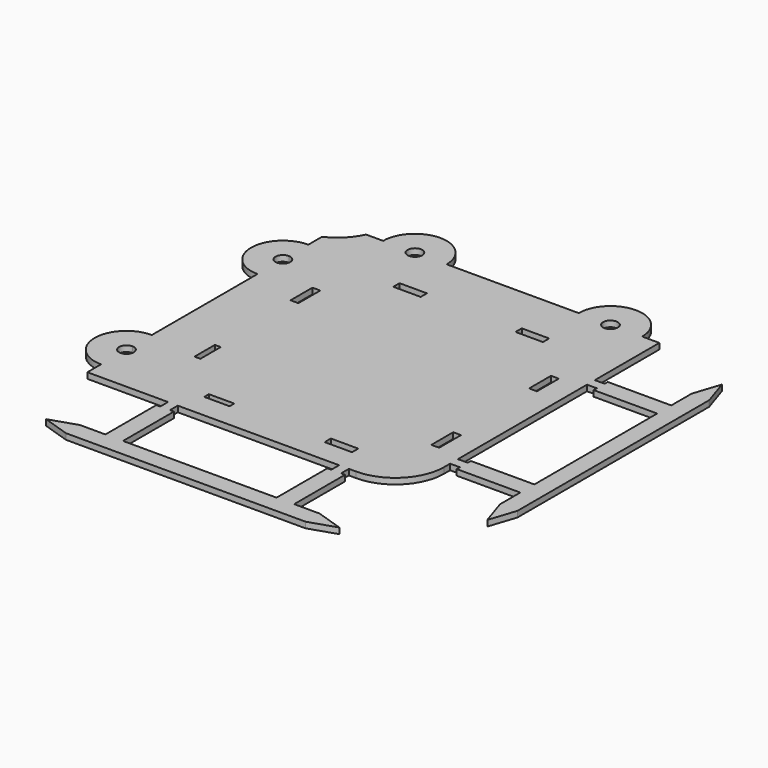
from build123d import *

# Parameters (mm, degrees)
F0_R        = 1.905
F0_W        = 2.032
F0_H        = 7.112
F0_W_2      = 7.112
F0_H_2      = 2.032
F0_W_3      = 2.54
F0_H_3      = 2.54
F0_W_4      = 6.604
F0_H_4      = 1.524
F0_W_5      = 1.524
F0_H_5      = 6.604
F1_DEPTH    = 1.524
F2_T1_DEPTH = 1.524
F2_T3_DEPTH = 65.024


# Not quite as in the source:
# - a fillet or chamfer that OpenCascade refuses, or shapes differently, is made with other operations: its cross-section is extruded or revolved along the edge and cut away or added


with BuildPart() as f1:
    # F0 (on Top) → F1 (new body)
    with BuildSketch(Plane.XY):
        with BuildLine():
            Line((38.1, 23.495), (38.1, 38.1))
            Line((38.1, 38.1), (30.674706153, 38.1))
            ThreePointArc((30.674706153, 38.1), (25.4, 36.195), (20.125293847, 38.1))
            Line((20.125293847, 38.1), (-20.125293847, 38.1))
            ThreePointArc((-20.125293847, 38.1), (-25.4, 36.195), (-30.674706153, 38.1))
            Line((-30.674706153, 38.1), (-38.1, 38.1))
            Line((-38.1, 38.1), (-38.1, 30.674706153))
            ThreePointArc((-38.1, 30.674706153), (-36.6858427695, 28.2040840751), (-36.195, 25.4))
            ThreePointArc((-36.195, 25.4), (-36.6858427695, 22.5959159249), (-38.1, 20.125293847))
            Line((-38.1, 20.125293847), (-38.1, -20.125293847))
            ThreePointArc((-38.1, -20.125293847), (-36.6858427695, -22.5959159249), (-36.195, -25.4))
            ThreePointArc((-36.195, -25.4), (-36.6858427695, -28.2040840751), (-38.1, -30.674706153))
            Line((-38.1, -30.674706153), (-38.1, -38.1))
            Line((-38.1, -38.1), (-23.495, -38.1))
            Line((-23.495, -38.1), (-20.955, -38.1))
            Line((-20.955, -38.1), (20.955, -38.1))
            Line((20.955, -38.1), (23.495, -38.1))
            Line((23.495, -38.1), (38.1, -38.1))
            Line((38.1, -38.1), (38.1, -23.495))
            Line((38.1, -23.495), (38.1, -20.955))
            Line((38.1, -20.955), (38.1, 20.955))
            Line((38.1, 20.955), (38.1, 23.495))
        make_face()
        with Locations((-25.4, -25.4)):
            Circle(F0_R, mode=Mode.SUBTRACT)
        with Locations((-30.988, -15.875)):
            Rectangle(F0_W, F0_H, mode=Mode.SUBTRACT)
        with Locations((-15.875, -30.988)):
            Rectangle(F0_W_2, F0_H_2, mode=Mode.SUBTRACT)
        with Locations((15.875, -30.988)):
            Rectangle(F0_W_2, F0_H_2, mode=Mode.SUBTRACT)
        with Locations((25.4, -25.4)):
            Circle(F0_R, mode=Mode.SUBTRACT)
        with Locations((30.988, -15.875)):
            Rectangle(F0_W, F0_H, mode=Mode.SUBTRACT)
        with Locations((-30.988, 15.875)):
            Rectangle(F0_W, F0_H, mode=Mode.SUBTRACT)
        with Locations((-25.4, 25.4)):
            Circle(F0_R, mode=Mode.SUBTRACT)
        with Locations((-15.875, 30.988)):
            Rectangle(F0_W_2, F0_H_2, mode=Mode.SUBTRACT)
        with Locations((30.988, 15.875)):
            Rectangle(F0_W, F0_H, mode=Mode.SUBTRACT)
        with Locations((15.875, 30.988)):
            Rectangle(F0_W_2, F0_H_2, mode=Mode.SUBTRACT)
        with Locations((25.4, 25.4)):
            Circle(F0_R, mode=Mode.SUBTRACT)
        Polygon((31.1238057911, -57.15), (24.511, -57.15), (19.939, -57.15), (0, -57.15), (-19.939, -57.15), (-24.511, -57.15), (-31.1238057911, -57.15), (-38.1, -59.436), (-31.1238057911, -61.722), (0, -61.722), (31.1238057911, -61.722), (38.1, -59.436), align=None)
        Polygon((-19.939, -40.64), (-20.955, -40.64), (-23.495, -40.64), (-24.511, -40.64), (-24.511, -57.15), (-19.939, -57.15), align=None)
        Polygon((24.511, -40.64), (23.495, -40.64), (20.955, -40.64), (19.939, -40.64), (19.939, -57.15), (24.511, -57.15), align=None)
        with Locations((22.225, -39.37)):
            Rectangle(F0_W_3, F0_H_3)
        with BuildLine():
            Line((-44.45, 27.305), (-44.45, 33.655))
            ThreePointArc((-44.45, 33.655), (-52.705, 25.4), (-44.45, 17.145))
            Line((-44.45, 17.145), (-44.45, 23.495))
            ThreePointArc((-44.45, 23.495), (-46.355, 25.4), (-44.45, 27.305))
        make_face()
        with BuildLine():
            Line((-44.45, -23.495), (-44.45, -17.145))
            ThreePointArc((-44.45, -17.145), (-52.705, -25.4), (-44.45, -33.655))
            Line((-44.45, -33.655), (-44.45, -27.305))
            ThreePointArc((-44.45, -27.305), (-46.355, -25.4), (-44.45, -23.495))
        make_face()
        with BuildLine():
            Line((-38.1, 20.125293847), (-38.1, 30.674706153))
            ThreePointArc((-38.1, 30.674706153), (-40.9426986366, 32.8728750924), (-44.45, 33.655))
            Line((-44.45, 33.655), (-44.45, 27.305))
            ThreePointArc((-44.45, 27.305), (-43.1029615818, 26.7470384182), (-42.545, 25.4))
            ThreePointArc((-42.545, 25.4), (-43.1029615818, 24.0529615818), (-44.45, 23.495))
            Line((-44.45, 23.495), (-44.45, 17.145))
            ThreePointArc((-44.45, 17.145), (-40.9426986366, 17.9271249076), (-38.1, 20.125293847))
        make_face()
        with BuildLine():
            Line((-38.1, 30.674706153), (-38.1, 38.1))
            Line((-38.1, 38.1), (-44.45, 38.1))
            Line((-44.45, 38.1), (-44.45, 33.655))
            ThreePointArc((-44.45, 33.655), (-40.9426986366, 32.8728750924), (-38.1, 30.674706153))
        make_face()
        with BuildLine():
            Line((-38.1, -38.1), (-38.1, -30.674706153))
            ThreePointArc((-38.1, -30.674706153), (-40.9426986366, -32.8728750924), (-44.45, -33.655))
            Line((-44.45, -33.655), (-44.45, -38.1))
            Line((-44.45, -38.1), (-38.1, -38.1))
        make_face()
        with BuildLine():
            Line((-38.1, -20.125293847), (-38.1, 20.125293847))
            ThreePointArc((-38.1, 20.125293847), (-40.9426986366, 17.9271249076), (-44.45, 17.145))
            Line((-44.45, 17.145), (-44.45, -17.145))
            ThreePointArc((-44.45, -17.145), (-40.9426986366, -17.9271249076), (-38.1, -20.125293847))
        make_face()
        with Locations((39.37, 22.225)):
            Rectangle(F0_W_3, F0_H_3)
        Polygon((40.64, 24.511), (40.64, 23.495), (40.64, 20.955), (40.64, 19.939), (57.15, 19.939), (57.15, 24.511), align=None)
        Polygon((57.15, 31.1238057911), (57.15, 24.511), (57.15, 19.939), (57.15, 0), (57.15, -19.939), (57.15, -24.511), (57.15, -31.1238057911), (59.436, -38.1), (61.722, -31.1238057911), (61.722, 0), (61.722, 31.1238057911), (59.436, 38.1), align=None)
        Polygon((40.64, -19.939), (40.64, -20.955), (40.64, -23.495), (40.64, -24.511), (57.15, -24.511), (57.15, -19.939), align=None)
        with Locations((39.37, -22.225)):
            Rectangle(F0_W_3, F0_H_3)
        with Locations((-22.225, -39.37)):
            Rectangle(F0_W_3, F0_H_3)
        with BuildLine():
            Line((-30.674706153, 38.1), (-20.125293847, 38.1))
            ThreePointArc((-20.125293847, 38.1), (-17.9271249076, 40.9426986366), (-17.145, 44.45))
            Line((-17.145, 44.45), (-23.495, 44.45))
            ThreePointArc((-23.495, 44.45), (-25.4, 42.545), (-27.305, 44.45))
            Line((-27.305, 44.45), (-33.655, 44.45))
            ThreePointArc((-33.655, 44.45), (-32.8728750924, 40.9426986366), (-30.674706153, 38.1))
        make_face()
        with BuildLine():
            ThreePointArc((-36.195, -25.4), (-36.6858427695, -22.5959159249), (-38.1, -20.125293847))
            Line((-38.1, -20.125293847), (-38.1, -30.674706153))
            ThreePointArc((-38.1, -30.674706153), (-36.6858427695, -28.2040840751), (-36.195, -25.4))
        make_face()
        with BuildLine():
            ThreePointArc((-30.674706153, 38.1), (-25.4, 36.195), (-20.125293847, 38.1))
            Line((-20.125293847, 38.1), (-30.674706153, 38.1))
        make_face()
        with BuildLine():
            Line((-23.495, 44.45), (-17.145, 44.45))
            ThreePointArc((-17.145, 44.45), (-25.4, 52.705), (-33.655, 44.45))
            Line((-33.655, 44.45), (-27.305, 44.45))
            ThreePointArc((-27.305, 44.45), (-25.4, 46.355), (-23.495, 44.45))
        make_face()
        with BuildLine():
            Line((-38.1, 38.1), (-30.674706153, 38.1))
            ThreePointArc((-30.674706153, 38.1), (-32.8728750924, 40.9426986366), (-33.655, 44.45))
            Line((-33.655, 44.45), (-38.1, 44.45))
            Line((-38.1, 44.45), (-38.1, 38.1))
        make_face()
        with BuildLine():
            Line((30.674706153, 38.1), (38.1, 38.1))
            Line((38.1, 38.1), (38.1, 44.45))
            Line((38.1, 44.45), (33.655, 44.45))
            ThreePointArc((33.655, 44.45), (32.8728750924, 40.9426986366), (30.674706153, 38.1))
        make_face()
        with BuildLine():
            Line((-38.1, -30.674706153), (-38.1, -20.125293847))
            ThreePointArc((-38.1, -20.125293847), (-40.9426986366, -17.9271249076), (-44.45, -17.145))
            Line((-44.45, -17.145), (-44.45, -23.495))
            ThreePointArc((-44.45, -23.495), (-43.1029615818, -24.0529615818), (-42.545, -25.4))
            ThreePointArc((-42.545, -25.4), (-43.1029615818, -26.7470384182), (-44.45, -27.305))
            Line((-44.45, -27.305), (-44.45, -33.655))
            ThreePointArc((-44.45, -33.655), (-40.9426986366, -32.8728750924), (-38.1, -30.674706153))
        make_face()
        with BuildLine():
            ThreePointArc((-36.195, 25.4), (-36.6858427695, 28.2040840751), (-38.1, 30.674706153))
            Line((-38.1, 30.674706153), (-38.1, 20.125293847))
            ThreePointArc((-38.1, 20.125293847), (-36.6858427695, 22.5959159249), (-36.195, 25.4))
        make_face()
        with BuildLine():
            Line((-20.125293847, 38.1), (20.125293847, 38.1))
            ThreePointArc((20.125293847, 38.1), (17.9271249076, 40.9426986366), (17.145, 44.45))
            Line((17.145, 44.45), (-17.145, 44.45))
            ThreePointArc((-17.145, 44.45), (-17.9271249076, 40.9426986366), (-20.125293847, 38.1))
        make_face()
        with BuildLine():
            Line((27.305, 44.45), (33.655, 44.45))
            ThreePointArc((33.655, 44.45), (25.4, 52.705), (17.145, 44.45))
            Line((17.145, 44.45), (23.495, 44.45))
            ThreePointArc((23.495, 44.45), (25.4, 46.355), (27.305, 44.45))
        make_face()
        with BuildLine():
            Line((20.125293847, 38.1), (30.674706153, 38.1))
            ThreePointArc((30.674706153, 38.1), (32.8728750924, 40.9426986366), (33.655, 44.45))
            Line((33.655, 44.45), (27.305, 44.45))
            ThreePointArc((27.305, 44.45), (25.4, 42.545), (23.495, 44.45))
            Line((23.495, 44.45), (17.145, 44.45))
            ThreePointArc((17.145, 44.45), (17.9271249076, 40.9426986366), (20.125293847, 38.1))
        make_face()
        with BuildLine():
            ThreePointArc((20.125293847, 38.1), (25.4, 36.195), (30.674706153, 38.1))
            Line((30.674706153, 38.1), (20.125293847, 38.1))
        make_face()
        with Locations((-25.4, 25.4)):
            Circle(F0_R)
        with Locations((-25.4, -25.4)):
            Circle(F0_R)
        with Locations((25.4, 25.4)):
            Circle(F0_R)
        with Locations((25.4, -25.4)):
            Circle(F0_R)
        with Locations((-15.875, -30.988)):
            Rectangle(F0_W_2, F0_H_2)
        with Locations((-15.875, -30.988)):
            Rectangle(F0_W_4, F0_H_4, mode=Mode.SUBTRACT)
        with Locations((-30.988, -15.875)):
            Rectangle(F0_W, F0_H)
        with Locations((-30.988, -15.875)):
            Rectangle(F0_W_5, F0_H_5, mode=Mode.SUBTRACT)
    extrude(amount=F1_DEPTH)

    # F2: fillet of radius 12.7 on 2 edges, made by hand

    # F2_s2 → F2_t1 (join)
    with BuildSketch(Plane.XY):
        with BuildLine():
            ThreePointArc((-38.1, 44.45), (-40.6950042916, 40.6950042916), (-44.45, 38.1))
            Line((-44.45, 38.1), (-38.1, 38.1))
            Line((-38.1, 38.1), (-38.1, 44.45))
        make_face()
    extrude(amount=F2_T1_DEPTH)

    # F2_s4 → F2_t3 (cut)
    with BuildSketch(Plane.XY.offset(-31.75)):
        with BuildLine():
            ThreePointArc((25.4, -38.1), (34.3802561211, -34.3802561211), (38.1, -25.4))
            Line((38.1, -25.4), (38.1, -38.1))
            Line((38.1, -38.1), (25.4, -38.1))
        make_face()
    extrude(amount=F2_T3_DEPTH, mode=Mode.SUBTRACT)


solid = f1.part
